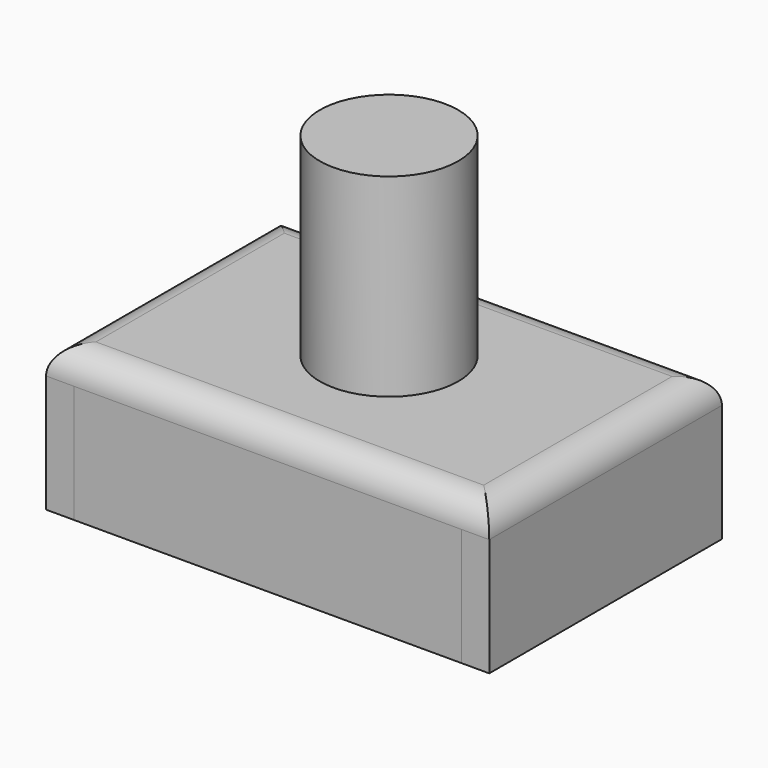
from build123d import *

# Parameters (mm, degrees)
F0_W      = 18
F0_H      = 17
F0_W_2    = 14
F0_H_2    = 13
F1_DEPTH  = 8
F2_W      = 9
F2_H      = 13
F3_DEPTH  = 2
F5_W      = 13
F5_H      = 12
F6_DEPTH  = 6
F7_R      = 3.5
F8_DEPTH  = 5
F9_R      = 3
F10_DEPTH = 10
F11_W     = 5
F11_H     = 17
F12_DEPTH = 2
F13_W     = 5
F13_H     = 4
F14_DEPTH = 6
F15_W     = 28
F15_H     = 8.5
F16_DEPTH = 2
F17_W     = 21
F17_H     = 8.5
F18_DEPTH = 2
F19_W     = 28
F19_H     = 8.5
F20_DEPTH = 2
F21_W     = 21
F21_H     = 8.5
F22_DEPTH = 2
F23_R     = 1.15
F24_DEPTH = 5
F25_W     = 32
F25_H     = 21
F26_DEPTH = 2
F27_R     = 3.75
F28_DEPTH = 5
F29_R     = 5
F30_DEPTH = 14
F31_R     = 1.99999


# Not quite as in the source:
# - a fillet or chamfer is up to 0.001 mm smaller than in the source, because OpenCascade refuses the exact size


with BuildPart() as f1:
    # F0 (on Top) → F1 (new body)
    with BuildSketch(Plane.XY):
        with Locations((7, -6.5)):
            Rectangle(F0_W, F0_H)
        with Locations((7, -6.5)):
            Rectangle(F0_W_2, F0_H_2, mode=Mode.SUBTRACT)
    extrude(amount=F1_DEPTH)

    # F2 (on face) → F3 (join)
    with BuildSketch(Plane(origin=(0, 0, 0), x_dir=(1, 0, 0), z_dir=(0, 0, -1))):
        with Locations((7, 6.5)):
            Rectangle(F2_W, F2_H)
    extrude(amount=-F3_DEPTH)

    # F11 (on Top) → F12 (join)
    with BuildSketch(Plane.XY):
        with Locations((-4.5, -6.5)):
            Rectangle(F11_W, F11_H)
        with Locations((18.5, -6.5)):
            Rectangle(F11_W, F11_H)
    extrude(amount=F12_DEPTH)

    # F13 (on face) → F14 (join)
    with BuildSketch(Plane.XY.offset(2)):
        with Locations((-4.5, -6.5)):
            Rectangle(F13_W, F13_H)
        with Locations((18.5, -6.5)):
            Rectangle(F13_W, F13_H)
    extrude(amount=F14_DEPTH)


with BuildPart() as f6:
    # F5 (on face) → F6 (new body)
    with BuildSketch(Plane.XY.offset(2)):
        with Locations((6.9626439363, -6.4136818983)):
            Rectangle(F5_W, F5_H)
    extrude(amount=F6_DEPTH)


with BuildPart() as f8:
    # F7 (on face) → F8 (new body)
    with BuildSketch(Plane.XY.offset(8)):
        with Locations((6.9626439363, -6)):
            Circle(F7_R)
    extrude(amount=F8_DEPTH)


with BuildPart() as f10:
    # F9 (on face) → F10 (new body)
    with BuildSketch(Plane.XY.offset(13)):
        with Locations((6.9626439363, -6)):
            Circle(F9_R)
    extrude(amount=F10_DEPTH)


with BuildPart() as f16:
    # F15 (on face) → F16 (new body)
    with BuildSketch(Plane.XZ.offset(15)):
        with Locations((7, 4.25)):
            Rectangle(F15_W, F15_H)
    extrude(amount=F16_DEPTH)


with BuildPart() as f18:
    # F17 (on face) → F18 (new body)
    with BuildSketch(Plane.YZ.offset(21)):
        with Locations((-6.5, 4.25)):
            Rectangle(F17_W, F17_H)
    extrude(amount=F18_DEPTH)


with BuildPart() as f20:
    # F19 (on face) → F20 (new body)
    with BuildSketch(Plane(origin=(0, 2, 0), x_dir=(-1, 0, 0), z_dir=(0, 1, 0))):
        with Locations((-7, 4.25)):
            Rectangle(F19_W, F19_H)
    extrude(amount=F20_DEPTH)


with BuildPart() as f22:
    # F21 (on face) → F22 (new body)
    with BuildSketch(Plane(origin=(-7, 0, 0), x_dir=(0, -1, 0), z_dir=(-1, 0, 0))):
        with Locations((6.5, 4.25)):
            Rectangle(F21_W, F21_H)
    extrude(amount=F22_DEPTH)


with BuildPart() as f24_tool:
    # F23 (on face) → F24 (new body)
    with BuildSketch(Plane(origin=(-9, 0, 0), x_dir=(0, -1, 0), z_dir=(-1, 0, 0))):
        with Locations((6.5, 4.85)):
            Circle(F23_R)
    extrude(amount=-F24_DEPTH)


with BuildPart() as f1_1:
    add(f1.part)

    # F24: cut by f24_tool
    add(f24_tool.part, mode=Mode.SUBTRACT)


with BuildPart() as f22_1:
    add(f22.part)

    # F24: cut by f24_tool
    add(f24_tool.part, mode=Mode.SUBTRACT)


with BuildPart() as f26:
    # F25 (on face) → F26 (new body)
    with BuildSketch(Plane.XY.offset(8.5)):
        with Locations((7, -6.5)):
            Rectangle(F25_W, F25_H)
    extrude(amount=F26_DEPTH)

    # F27 (on face) → F28 (cut)
    with BuildSketch(Plane.XY.offset(13)):
        with Locations((6.9626439363, -6)):
            Circle(F27_R)
    extrude(amount=-F28_DEPTH, mode=Mode.SUBTRACT)

    # F31 (radius 2 in the source; OpenCascade refuses exactly that, so slightly less here)
    f31_edges = [f26.edges().sort_by_distance(p)[0] for p in [
        (-9, -6.5, 10.5),
        (7, 4, 10.5),
        (7, -17, 10.5),
        (23, -6.5, 10.5),
    ]]
    fillet(f31_edges, radius=F31_R)


with BuildPart() as f30:
    # F29 (on face) → F30 (new body)
    with BuildSketch(Plane.XY.offset(10.5)):
        with Locations((6.9626439363, -6)):
            Circle(F29_R)
    extrude(amount=F30_DEPTH)


solid = Compound([f6.part, f8.part, f10.part, f16.part, f18.part, f20.part, f1_1.part, f22_1.part, f26.part, f30.part])
